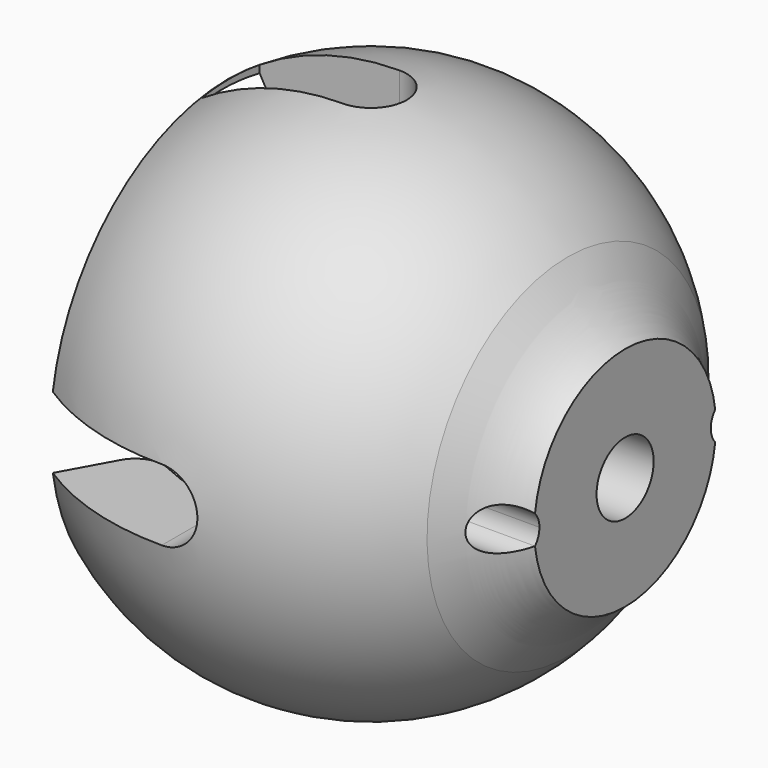
from build123d import *

# Parameters (mm, degrees)
F2_R     = 2
F4_DEPTH = 27.8020402442
F3_R     = 1.5
F3_R_2   = 2.5
F5_DEPTH = 27.8020402442
F7_DEPTH = 25
F9_DEPTH = 25


with BuildPart() as f1:
    # F0 (on Front) → F1 (revolve)
    with BuildSketch(Plane.XZ):
        with BuildLine():
            ThreePointArc((-7.0685046336, 10.3095219212), (5.4017622611, 11.2725757693), (12.4638702008, 0.949705016))
            Line((12.4638702008, 0.949705016), (17.7978035063, 0.949705016))
            Line((17.7978035063, 0.949705016), (17.7978035063, 7.949705016))
            add(Edge.make_bspline(
                [(13.7809895682, 12.3177978136), (15.1477944904, 10.0637607805), (16.4248201761, 8.7362514946), (17.7978035063, 7.949705016)],
                knots=[0, 0, 0, 0, 0.1514236362, 0.1514236362, 0.1514236362, 0.1514236362], degree=3))
            ThreePointArc((13.7809895682, 12.3177978136), (2.4835532955, 18.3159979112), (-10.003236638, 15.5428141988))
            Line((-10.003236638, 15.5428141988), (-7.0685046336, 10.3095219212))
        make_face()
    revolve(axis=Axis((35, 0, 0), (1, 0, 0)))

    # F2
    f2_edges = [f1.edges().sort_by_distance(p)[0] for p in [
        (-7.068505, 0, -10.309522),
    ]]
    fillet(f2_edges, radius=F2_R)

    # F3 (on face) → F4 (cut, through all)
    with BuildSketch(Plane.YZ.offset(17.7978035063)):
        with BuildLine():
            ThreePointArc((-7.8859894356, -1.0044801951), (-7.949705016, 0), (-7.8859894356, 1.0044801951))
            ThreePointArc((-7.8859894356, 1.0044801951), (-10.5, 0), (-7.8859894356, -1.0044801951))
        make_face()
        with BuildLine():
            ThreePointArc((7.949705016, 0), (7.9337601304, 0.5032494753), (7.8859894356, 1.0044801951))
            ThreePointArc((7.8859894356, 1.0044801951), (7.5, 0), (7.8859894356, -1.0044801951))
            ThreePointArc((7.8859894356, -1.0044801951), (7.9337601304, -0.5032494753), (7.949705016, 0))
        make_face()
        with BuildLine():
            ThreePointArc((10.5, 0), (9.5380446791, 1.4001813894), (7.8859894356, 1.0044801951))
            ThreePointArc((7.8859894356, 1.0044801951), (7.9337601304, 0.5032494753), (7.949705016, 0))
            ThreePointArc((7.949705016, 0), (7.9337601304, -0.5032494753), (7.8859894356, -1.0044801951))
            ThreePointArc((7.8859894356, -1.0044801951), (9.5380446791, -1.4001813894), (10.5, 0))
        make_face()
        with BuildLine():
            ThreePointArc((-7.8859894356, -1.0044801951), (-7.5998186106, -0.5380446791), (-7.5, 0))
            ThreePointArc((-7.5, 0), (-7.5998186106, 0.5380446791), (-7.8859894356, 1.0044801951))
            ThreePointArc((-7.8859894356, 1.0044801951), (-7.949705016, 0), (-7.8859894356, -1.0044801951))
        make_face()
    extrude(amount=-F4_DEPTH, mode=Mode.SUBTRACT)

    # F3 (on face) → F5 (cut, through all)
    with BuildSketch(Plane.YZ.offset(17.7978035063)):
        with Locations((-9, 0)):
            Circle(F3_R)
        with Locations((9, 0)):
            Circle(F3_R)
        Circle(F3_R_2)
    extrude(amount=-F5_DEPTH, mode=Mode.SUBTRACT)

    # F6 (on Front) → F7 (cut, symmetric)
    with BuildSketch(Plane.XZ):
        with BuildLine():
            Line((-10.1115526631, -2.5), (0, -2.5))
            ThreePointArc((0, -2.5), (2.5, 0), (0, 2.5))
            Line((0, 2.5), (-10.1115526631, 2.5))
            Line((-10.1115526631, 2.5), (-10.1115526631, -2.5))
        make_face()
    extrude(amount=F7_DEPTH, both=True, mode=Mode.SUBTRACT)

    # F8 (on Top) → F9 (cut, symmetric)
    with BuildSketch(Plane.XY):
        with BuildLine():
            Line((-9.8809963092, -2.5), (0, -2.5))
            ThreePointArc((0, -2.5), (2.5, 0), (0, 2.5))
            Line((0, 2.5), (-9.7886603326, 2.5))
            Line((-9.7886603326, 2.5), (-9.8809963092, -2.5))
        make_face()
    extrude(amount=F9_DEPTH, both=True, mode=Mode.SUBTRACT)


solid = f1.part
